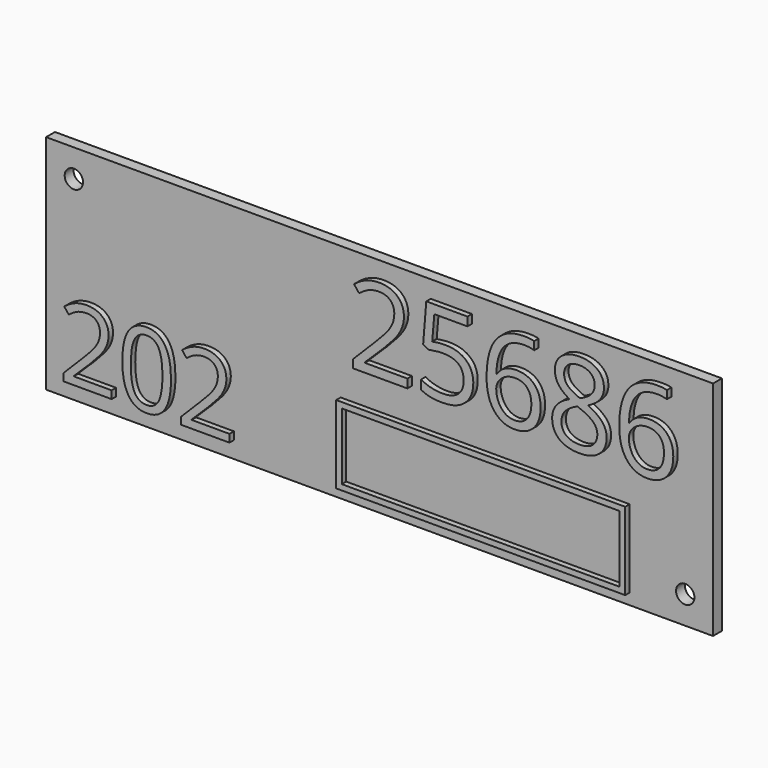
from build123d import *

# Parameters (mm, degrees)
F0_W         = 120
F0_H         = 40
F1_DEPTH     = 2
F3_D         = 3.3
F4_TEXT_SIZE = 20.871833895
F5_DEPTH     = 1
F6_TEXT_SIZE = 18.5356140827
F7_DEPTH     = 1
F8_W         = 52
F8_H         = 14
F8_W_2       = 49.99999962
F8_H_2       = 11.99999962
F9_DEPTH     = 1


# Not quite as in the source:
# - Text() gives the source's letters only with a copy of the font that has no kerning and outlines rounded to 1/6400 em; it was checked with that copy


with BuildPart() as f1:
    # F0 (on Front) → F1 (new body)
    with BuildSketch(Plane.XZ):
        Rectangle(F0_W, F0_H)
    extrude(amount=F1_DEPTH)

    # F3 (through all)
    with Locations(Plane.XZ.offset(2)):
        with Locations((-55, 15), (55, -15)):
            Hole(F3_D / 2)

    # F4 (on face) → F5 (join)
    with BuildSketch(Plane.XZ.offset(2)):
        with Locations((-5, 2)):
            Text('25686', F4_TEXT_SIZE, font='Open Sans', text_align=(TextAlign.LEFT, TextAlign.BOTTOM))
    extrude(amount=F5_DEPTH)

    # F6 (on face) → F7 (join)
    with BuildSketch(Plane.XZ.offset(2)):
        with Locations((-57, -17)):
            Text('202', F6_TEXT_SIZE, font='Open Sans', text_align=(TextAlign.LEFT, TextAlign.BOTTOM))
    extrude(amount=F7_DEPTH)

    # F8 (on face) → F9 (join)
    with BuildSketch(Plane.XZ.offset(2)):
        with Locations((19, -11)):
            Rectangle(F8_W, F8_H)
        with Locations((19, -11)):
            Rectangle(F8_W_2, F8_H_2, mode=Mode.SUBTRACT)
    extrude(amount=F9_DEPTH)


solid = f1.part
